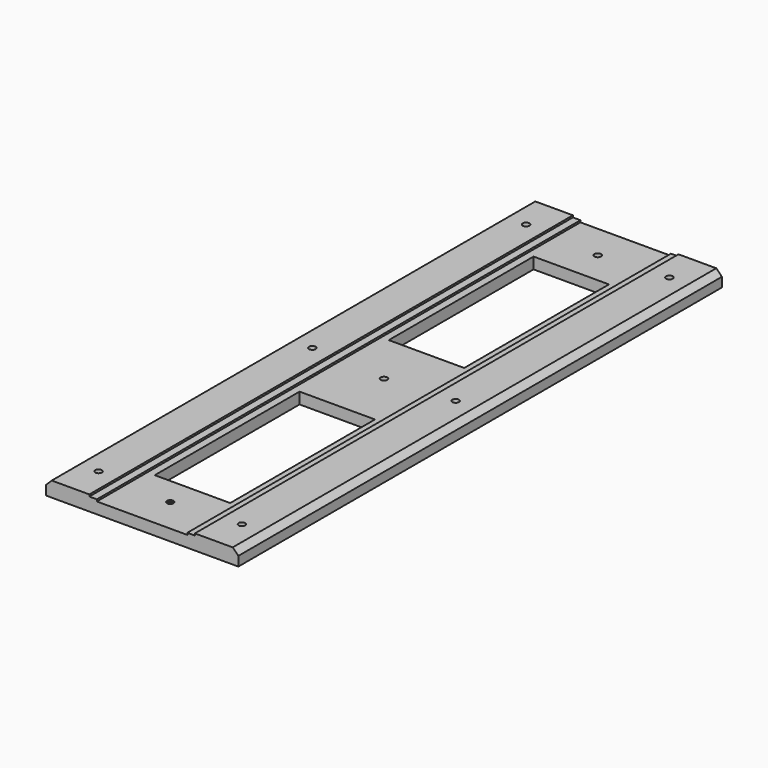
from build123d import *

# Parameters (mm, degrees)
F0_W                   = 323.799
F0_H                   = 1018.061
F0_W_2                 = 127
F0_H_2                 = 304.8
F1_DEPTH               = 25.4
F2_W                   = 177.8
F2_H                   = 1077.8446237831
F3_DEPTH               = 3.175
F4_W                   = 152.4
F4_H                   = 1094.5154423737
F5_DEPTH               = 3.175
F6_SIZE                = 9.525
F8_D                   = 6.6
F8_DEPTH               = 25
F8_CBORE_D             = 11.25
F8_CBORE_DEPTH         = 6
F8_TIP                 = 1.9828400428
F10_D                  = 6.6
F10_DEPTH              = 25
F10_CBORE_D            = 11.25
F10_CBORE_DEPTH        = 6
F10_TIP                = 1.9828400428
F13_D                  = 6.6
F13_CBORE_D            = 11.25
F13_CBORE_DEPTH        = 6
F13_ON_F12_D           = 6.6
F13_ON_F12_CBORE_D     = 11.25
F13_ON_F12_CBORE_DEPTH = 6


# Not quite as in the source:
# - a feature names something its author has since deleted; it is built from what else it names


with BuildPart() as f1:
    # F0 (on Top) → F1 (new body)
    with BuildSketch(Plane.XY):
        with Locations((-161.8995, 509.0305)):
            Rectangle(F0_W, F0_H)
        with Locations((-162.103, 258.488)):
            Rectangle(F0_W_2, F0_H_2, mode=Mode.SUBTRACT)
        with Locations((-162.103, 751.124)):
            Rectangle(F0_W_2, F0_H_2, mode=Mode.SUBTRACT)
    extrude(amount=F1_DEPTH)

    # F2 (on face) → F3 (cut)
    with BuildSketch(Plane.XY.offset(25.4)):
        with Locations((-162.103, 495.1518476009)):
            Rectangle(F2_W, F2_H)
    extrude(amount=-F3_DEPTH, mode=Mode.SUBTRACT)

    # F4 (on face) → F5 (cut)
    with BuildSketch(Plane.XY.offset(22.225)):
        with Locations((-162.103, 504.4111407595)):
            Rectangle(F4_W, F4_H)
    extrude(amount=-F5_DEPTH, mode=Mode.SUBTRACT)

    # F6
    f6_edges = [f1.edges().sort_by_distance(p)[0] for p in [
        (-323.799, 509.0305, 25.4),
        (0, 509.0305, 25.4),
    ]]
    chamfer(f6_edges, length=F6_SIZE)

    # F8
    with Locations(Plane.XY.offset(25.4)):
        with Locations((-41.16, 59.0305), (-41.16, 509.0305), (-41.16, 959.0305)):
            CounterBoreHole(F8_D / 2, F8_CBORE_D / 2, F8_CBORE_DEPTH, depth=F8_DEPTH)
            with Locations((0, 0, -(F8_DEPTH + F8_TIP / 2))):  # 118° drill point
                Cone(0, F8_D / 2, F8_TIP, mode=Mode.SUBTRACT)

    # F10
    with Locations(Plane.XY.offset(25.4)):
        with Locations((-282.6385, 59.0305), (-282.6385, 509.0305), (-282.6385, 959.0305)):
            CounterBoreHole(F10_D / 2, F10_CBORE_D / 2, F10_CBORE_DEPTH, depth=F10_DEPTH)
            with Locations((0, 0, -(F10_DEPTH + F10_TIP / 2))):  # 118° drill point
                Cone(0, F10_D / 2, F10_TIP, mode=Mode.SUBTRACT)

    # F13 (through all)
    with Locations(Plane.XY.offset(22.225)):
        with Locations((-161.89925, 59.0305)):
            CounterBoreHole(F13_D / 2, F13_CBORE_D / 2, F13_CBORE_DEPTH)

    # F13 on F12 (through all)
    with Locations(Plane.XY.offset(19.05)):
        with Locations((-161.89925, 509.0305), (-161.89925, 959.0305)):
            CounterBoreHole(F13_ON_F12_D / 2, F13_ON_F12_CBORE_D / 2, F13_ON_F12_CBORE_DEPTH)


solid = f1.part
